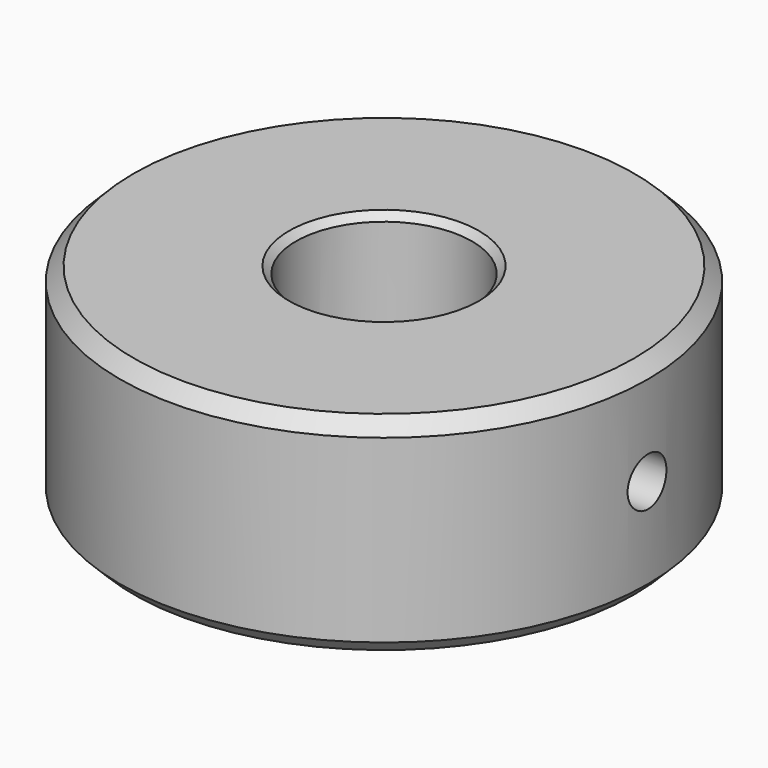
from build123d import *

# Parameters (mm, degrees)
F0_R           = 38.1
F0_R_2         = 12.7
F1_DEPTH       = 30
F2_SIZE        = 2
F4_D           = 7
F4_DEPTH       = 38.101
F5_D           = 7
F8_D           = 18
F8_DEPTH       = 10
F8_CBORE_D     = 25
F8_CBORE_DEPTH = 2
F8_TIP         = 5.4077455712
F9_SIZE        = 1


# Not quite as in the source:
# - a length typed as a fraction of an inch, garbled in the dataset ("3 / 203.2 mm" for 3/8 in), is restored


with BuildPart() as f1:
    # F0 (on Top) → F1 (new body)
    with BuildSketch(Plane.XY):
        Circle(F0_R)
        Circle(F0_R_2, mode=Mode.SUBTRACT)
    extrude(amount=F1_DEPTH)

    # F2
    f2_edges = [f1.edges().sort_by_distance(p)[0] for p in [
        (-38.1, 0, 30),
        (-38.1, 0, 0),
    ]]
    chamfer(f2_edges, length=F2_SIZE)

    # F4 (through all, one way)
    with BuildSketch(Plane(origin=(0, 0, 0), x_dir=(0, 1, 0), z_dir=(-1, 0, 0))):
        with Locations((0, -15)):
            Circle(F4_D / 2)
    extrude(amount=-F4_DEPTH, mode=Mode.SUBTRACT)

    # F5 (through all)
    with Locations(Plane.YZ):
        with Locations((0, 15)):
            Hole(F5_D / 2)

    # F8
    with Locations(Plane(origin=(-38.1, 0, 0), x_dir=(0, 1, 0), z_dir=(-1, 0, 0))):
        with Locations((0, -15.1190431789)):
            CounterBoreHole(F8_D / 2, F8_CBORE_D / 2, F8_CBORE_DEPTH, depth=F8_DEPTH)
            with Locations((0, 0, -(F8_DEPTH + F8_TIP / 2))):  # 118° drill point
                Cone(0, F8_D / 2, F8_TIP, mode=Mode.SUBTRACT)

    # F9
    f9_edges = [f1.edges().sort_by_distance(p)[0] for p in [
        (-12.7, 0, 0),
        (-12.7, 0, 30),
    ]]
    chamfer(f9_edges, length=F9_SIZE)


solid = f1.part
